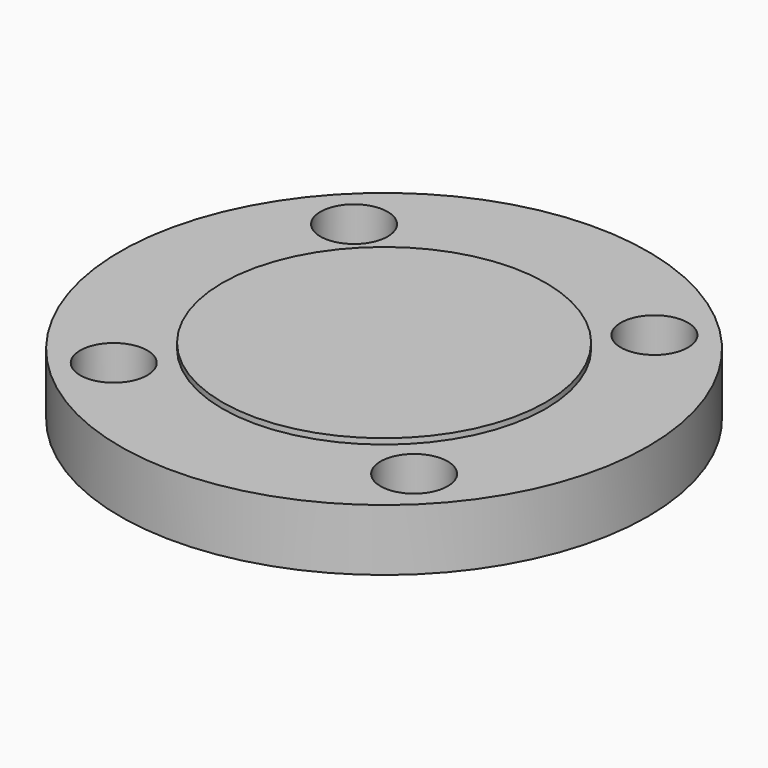
from build123d import *

# Parameters (mm, degrees)
F2_R     = 75
F2_R_2   = 9.55
F2_R_3   = 45.95
F4_DEPTH = 17.5
F5_DEPTH = 19.1


with BuildPart() as f4:
    # F2 (on Top) → F4 (new body)
    with BuildSketch(Plane.XY):
        Circle(F2_R)
        with Locations((-42.6738942446, -42.6738942446)):
            Circle(F2_R_2, mode=Mode.SUBTRACT)
        with Locations((42.6738942446, -42.6738942446)):
            Circle(F2_R_2, mode=Mode.SUBTRACT)
        with Locations((-42.6738942446, 42.6738942446)):
            Circle(F2_R_2, mode=Mode.SUBTRACT)
        Circle(F2_R_3, mode=Mode.SUBTRACT)
        with Locations((42.6738942446, 42.6738942446)):
            Circle(F2_R_2, mode=Mode.SUBTRACT)
    extrude(amount=F4_DEPTH)

    # F2 (on Top) → F5 (join)
    with BuildSketch(Plane.XY):
        Circle(F2_R_3)
    extrude(amount=F5_DEPTH)


solid = f4.part
